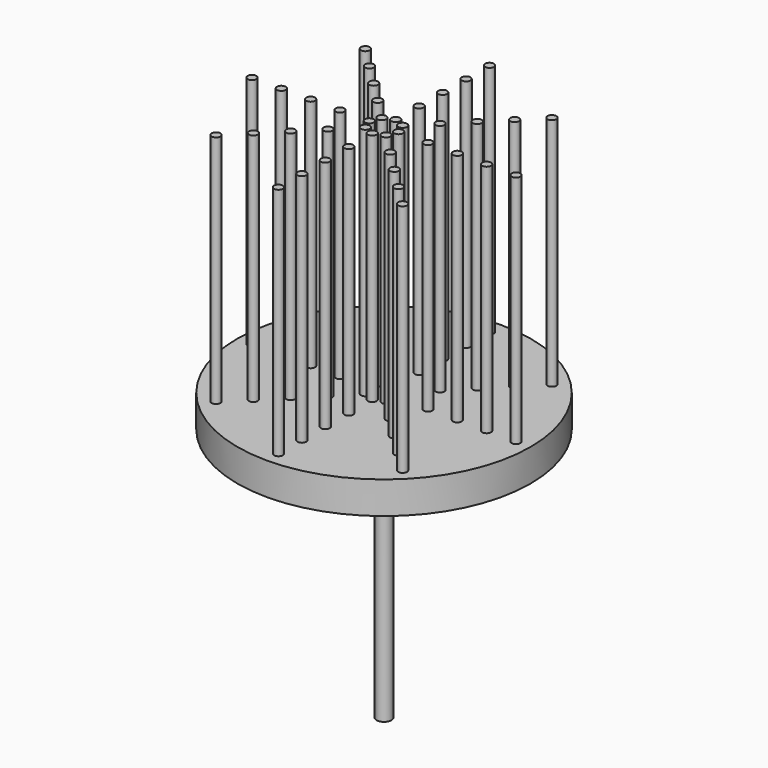
from build123d import *

# Parameters (mm, degrees)
F0_R            = 100
F1_DEPTH        = 22
F2_R            = 3
F3_DEPTH        = 160
F3_COPIES_COUNT = 8
F4_R            = 15
F5_DEPTH        = 23
F6_R            = 5
F7_DEPTH        = 150


# Not quite as in the source:
# - a pattern or mirror of a feature is missing from the dataset's text; its kind, count and spacing are read off the source's solid


with BuildPart() as f1:
    # F0 (on Top) → F1 (new body)
    with BuildSketch(Plane.XY):
        Circle(F0_R)
    extrude(amount=F1_DEPTH)

    # F2 (on face) → F3 (join)
    with BuildSketch(Plane.XY.offset(22)):
        with Locations((10, 0)):
            Circle(F2_R)
        with Locations((30, 0)):
            Circle(F2_R)
        with Locations((50, 0)):
            Circle(F2_R)
        with Locations((70, 0)):
            Circle(F2_R)
        with Locations((90, 0)):
            Circle(F2_R)
    f3 = extrude(amount=F3_DEPTH)

    # F3_copies: F3 ×8 about axis
    f3_copies_axis = Axis((0, 0, 0), (0, 0, 1))
    for i in range(1, F3_COPIES_COUNT):
        add(f3.rotate(f3_copies_axis, i * 360 / F3_COPIES_COUNT))

    # F4 (on face) → F5 (join)
    with BuildSketch(Plane.XY):
        Circle(F4_R)
    extrude(amount=-F5_DEPTH)

    # F6 (on face) → F7 (join)
    with BuildSketch(Plane(origin=(0, 0, -23), x_dir=(1, 0, 0), z_dir=(0, 0, -1))):
        Circle(F6_R)
    extrude(amount=F7_DEPTH)


solid = f1.part
